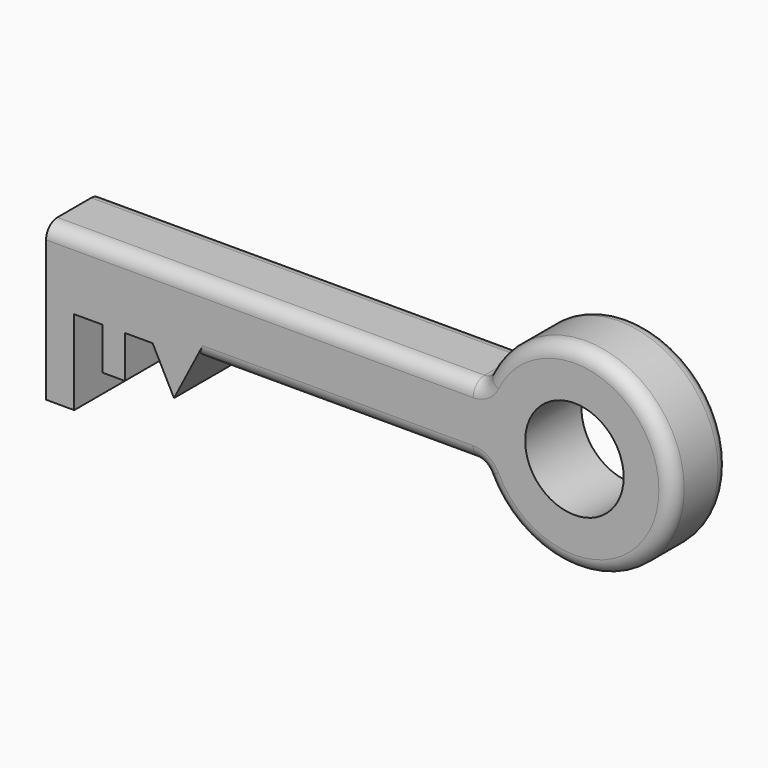
from build123d import *

# Parameters (mm, degrees)
F0_R     = 17.5
F0_W     = 10
F0_H     = 30
F0_W_2   = 8
F0_H_2   = 15
F1_DEPTH = 25
F2_F1_R  = 5
F2_F2_R  = 5


with BuildPart() as f1:
    # F0 (on Front) → F1 (new body)
    with BuildSketch(Plane.XZ):
        with BuildLine():
            Line((-76.905815019, -12.5), (25.0358718634, -12.5))
            ThreePointArc((25.0358718634, -12.5), (92.7276139399, 0), (25.0358718634, 12.5))
            Line((25.0358718634, 12.5), (-129.9641281366, 12.5))
            Line((-129.9641281366, 12.5), (-129.9641281366, -12.5))
            Line((-129.9641281366, -12.5), (-119.9641281366, -12.5))
            Line((-119.9641281366, -12.5), (-109.9641281366, -12.5))
            Line((-109.9641281366, -12.5), (-101.9641281366, -12.5))
            Line((-101.9641281366, -12.5), (-92.1254744445, -12.5))
            Line((-92.1254744445, -12.5), (-76.905815019, -12.5))
        make_face()
        with Locations((57.7276139399, 0)):
            Circle(F0_R, mode=Mode.SUBTRACT)
        with Locations((-124.9641281366, -27.5)):
            Rectangle(F0_W, F0_H)
        with Locations((-105.9641281366, -20)):
            Rectangle(F0_W_2, F0_H_2)
        Polygon((-84.5156447317, -27.2000782564), (-76.905815019, -12.5), (-92.1254744445, -12.5), align=None)
    extrude(amount=F1_DEPTH)

    # F2: fillet of radius 5 on 4 edges, made by hand

    # F2_f1
    f2_f1_edges = [f1.edges().sort_by_distance(p)[0] for p in [
        (25.0358718634, -12.5, -12.5),
        (25.0358718634, -12.5, 12.5),
    ]]
    fillet(f2_f1_edges, radius=F2_F1_R)

    # F2_f2
    f2_f2_edges = [f1.edges().sort_by_distance(p)[0] for p in [
        (92.7276139399, 0, 0),
        (92.7276139399, -25, 0),
        (24.4105279445, -25, -13.2610437605),
        (24.4105279445, -25, 13.2610437605),
        (24.4105279445, 0, -13.2610437605),
        (24.4105279445, 0, 13.2610437605),
    ]]
    fillet(f2_f2_edges, radius=F2_F2_R)


solid = f1.part
